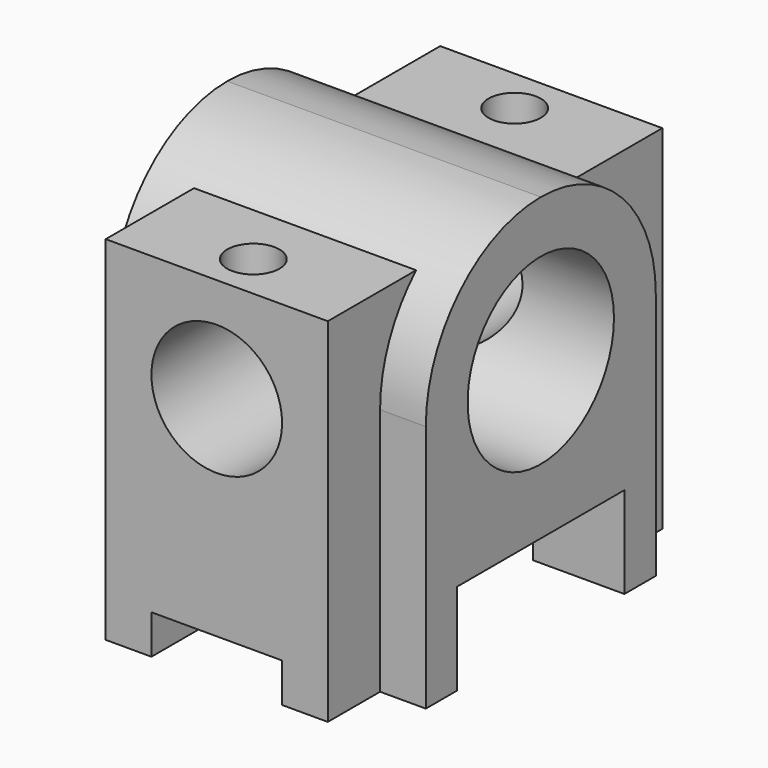
from build123d import *

# Parameters (mm, degrees)
F0_W          = 44
F0_H          = 60
F1_DEPTH      = 24
F2_R          = 21.99999
F3_W          = 34
F3_H          = 54
F4_DEPTH      = 10
F4_DEPTH_BACK = 54
F5_R          = 14
F5_W          = 32
F5_H          = 14
F6_DEPTH      = 48.001
F8_R          = 10
F8_W          = 20
F8_H          = 6
F9_DEPTH      = 64.001
F7_R          = 4
F10_DEPTH     = 7.8348487101


# Not quite as in the source:
# - a fillet or chamfer is up to 0.001 mm smaller than in the source, because OpenCascade refuses the exact size


with BuildPart() as f1:
    # F0 (on Right) → F1 (new body, symmetric)
    with BuildSketch(Plane.YZ):
        Rectangle(F0_W, F0_H)
    extrude(amount=F1_DEPTH, both=True)

    # F2 (radius 22 in the source; OpenCascade refuses exactly that, so slightly less here)
    f2_edges = [f1.edges().sort_by_distance(p)[0] for p in [
        (0, -22, 30),
        (0, 22, 30),
    ]]
    fillet(f2_edges, radius=F2_R)

    # F3 (on face) → F4 (join, two sides)
    with BuildSketch(Plane.XZ.offset(22)) as f4_sk:
        with Locations((0, -3)):
            Rectangle(F3_W, F3_H)
    extrude(amount=F4_DEPTH)
    extrude(f4_sk.sketch, amount=-F4_DEPTH_BACK)

    # F5 (on face) → F6 (cut, through all)
    with BuildSketch(Plane.YZ.offset(24)):
        with Locations((0, 8)):
            Circle(F5_R)
        with Locations((0, -23)):
            Rectangle(F5_W, F5_H)
    extrude(amount=-F6_DEPTH, mode=Mode.SUBTRACT)

    # F8 (on face) → F9 (cut, through all)
    with BuildSketch(Plane.XZ.offset(32)):
        with Locations((0, 8)):
            Circle(F8_R)
        with Locations((0, -27)):
            Rectangle(F8_W, F8_H)
    extrude(amount=-F9_DEPTH, mode=Mode.SUBTRACT)

    # F7 (on face) → F10 (cut, up to face)
    with BuildSketch(Plane.XY.offset(24)):
        with Locations((0, -25)):
            Circle(F7_R)
        with Locations((0, 25)):
            Circle(F7_R)
    extrude(amount=-F10_DEPTH, mode=Mode.SUBTRACT)


solid = f1.part
